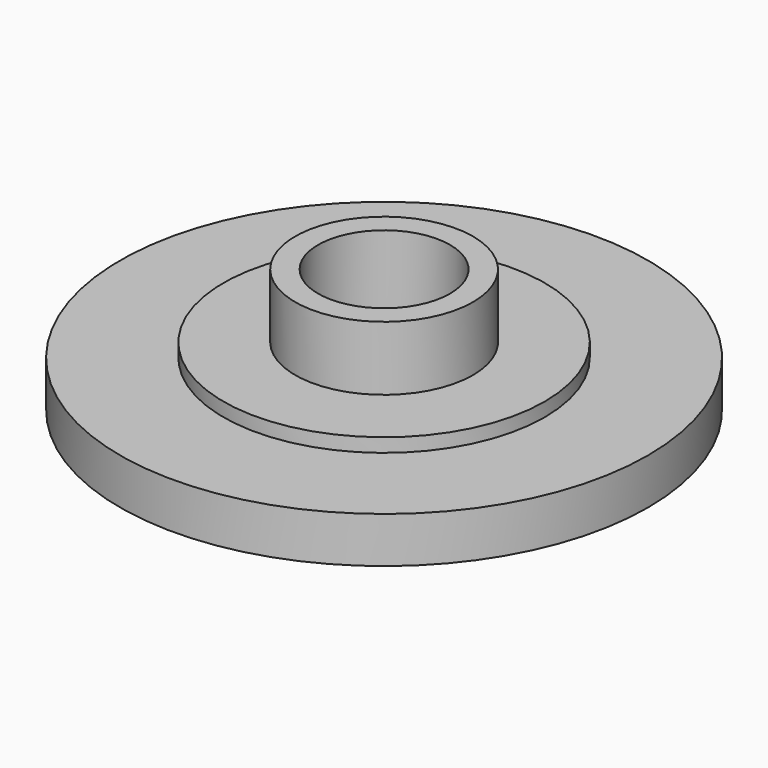
from build123d import *

# Parameters (mm, degrees)
F0_R     = 3.875
F1_DEPTH = 3.4
F0_R_2   = 7
F2_DEPTH = 0.6
F0_R_3   = 11.5
F3_DEPTH = 2
F4_T     = 1


# Not quite as in the source:
# - a shell that OpenCascade refuses in one call is made with other operations: the cavity is built on its own and cut out


with BuildPart() as f1:
    # F0 (on Top) → F1 (new body)
    with BuildSketch(Plane.XY):
        Circle(F0_R)
    extrude(amount=F1_DEPTH)

    # F0 (on Top) → F2 (join)
    with BuildSketch(Plane.XY):
        Circle(F0_R_2)
        Circle(F0_R, mode=Mode.SUBTRACT)
    extrude(amount=F2_DEPTH)

    # F0 (on Top) → F3 (join)
    with BuildSketch(Plane.XY):
        Circle(F0_R_3)
        Circle(F0_R_2, mode=Mode.SUBTRACT)
        Circle(F0_R_2)
        Circle(F0_R, mode=Mode.SUBTRACT)
        Circle(F0_R)
    extrude(amount=-F3_DEPTH)

    # F4: shell of thickness 1, made by hand


with BuildPart() as f4_core1:
    # F4_t2: copy of F1
    add(f1.part)

    # the walls: a layer under each face that stays
    f4_faces = [f4_core1.faces().sort_by_distance(p)[0] for p in [
        (-11.5, 0, -1),
        (-7.6666666667, -7.6666666667, 0),
        (0, 0, -2),
        (-7, 0, 0.3),
        (-4.6666666667, -4.6666666667, 0.6),
        (-3.875, 0, 2),
    ]]
    thicken(f4_faces, amount=-F4_T, mode=Mode.SUBTRACT)

    # F4_s3 → F4_t4 (revolve, cut)
    with BuildSketch(Plane.XZ):
        Polygon((7.01, 0.01), (7, -1), (6, -1), (6, 0), align=None)
    revolve(axis=Axis((0, 0, 0), (0, 0, 1)), mode=Mode.SUBTRACT)

    # F4_s5 → F4_t6 (revolve, cut)
    with BuildSketch(Plane.XZ):
        Polygon((3.885, 0.61), (3.875, -0.4), (2.875, -0.4), (2.875, 0.6), align=None)
    revolve(axis=Axis((0, 0, 0.6), (0, 0, 1)), mode=Mode.SUBTRACT)


with BuildPart() as f1_1:
    add(f1.part)

    # what is left inside the walls is the cavity
    f4_cavity = [f4_core1.part.solids().sort_by_distance(p)[0] for p in [
        (0, -2, -0.99),
    ]]
    add(f4_cavity, mode=Mode.SUBTRACT)


solid = f1_1.part
